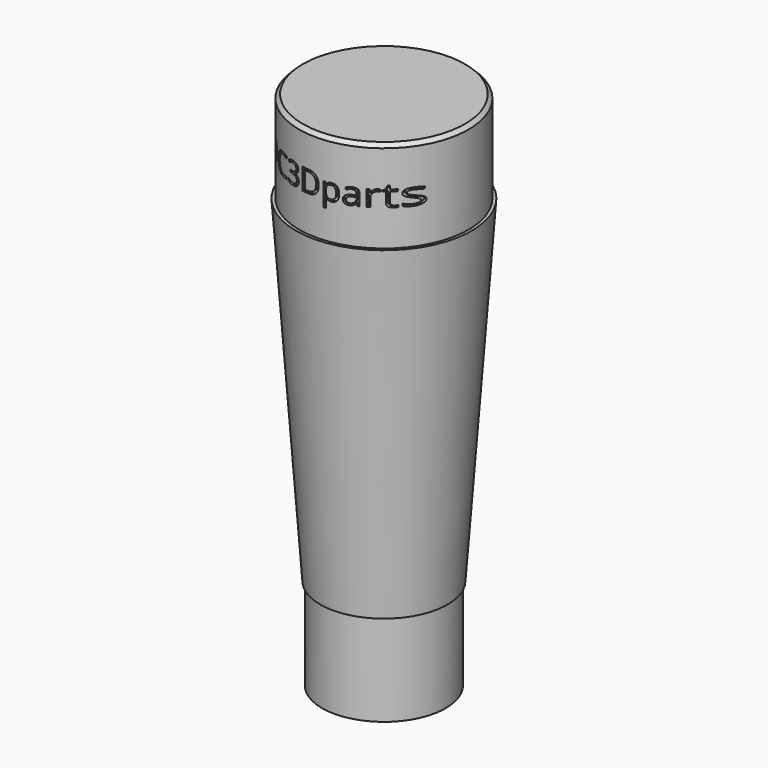
from build123d import *

# Parameters (mm, degrees)
F2_SIZE      = 1.2
F4_TEXT_SIZE = 9.7222222222
F5_DEPTH     = 35
F6_W         = 27
F6_H         = 27.6128641036


# Not quite as in the source:
# - Text() gives the source's letters only with a copy of the font that has no kerning and outlines rounded to 1/6400 em; it was checked with that copy


with BuildPart() as f1:
    # F0 (on Front) → F1 (revolve)
    with BuildSketch(Plane.XZ):
        Polygon((0, 73.2666279856), (-27.685, 73.2666279856), (-27.685, 43.2666279856), (-28.685, 43.2666279856), (-20.8, -66.7333720144), (-20.2, -66.7333720144), (-20.2, -96.7333720144), (0, -96.7333720144), align=None)
    revolve(axis=Axis((0, 0, -2.5966958965), (0, 0, -1)))

    # F2
    f2_edges = [f1.edges().sort_by_distance(p)[0] for p in [
        (27.685, 0, 73.266628),
    ]]
    chamfer(f2_edges, length=F2_SIZE)


with BuildPart() as f5:
    # F4 (on offset) → F5 (new body, through all)
    with BuildSketch(Plane.XZ.offset(35)):
        with Locations((-24.4146110883, 55.0184423855)):
            Text('DC3Dparts', F4_TEXT_SIZE, font='Open Sans', text_align=(TextAlign.LEFT, TextAlign.BOTTOM))
    extrude(amount=-F5_DEPTH)


with BuildPart() as f7:
    # F6 (on Front) → F7 (revolve)
    with BuildSketch(Plane.XZ):
        with Locations((-13.5, 62.5203610225)):
            Rectangle(F6_W, F6_H)
    revolve(axis=Axis((0, 0, 62.5203610225), (0, 0, 1)))


with BuildPart() as f5_1:
    add(f5.part)

    # F8: cut F7
    add(f7.part, mode=Mode.SUBTRACT)


with BuildPart() as f1_1:
    add(f1.part)

    # F9: cut F5
    add(f5_1.part, mode=Mode.SUBTRACT)


solid = f1_1.part
